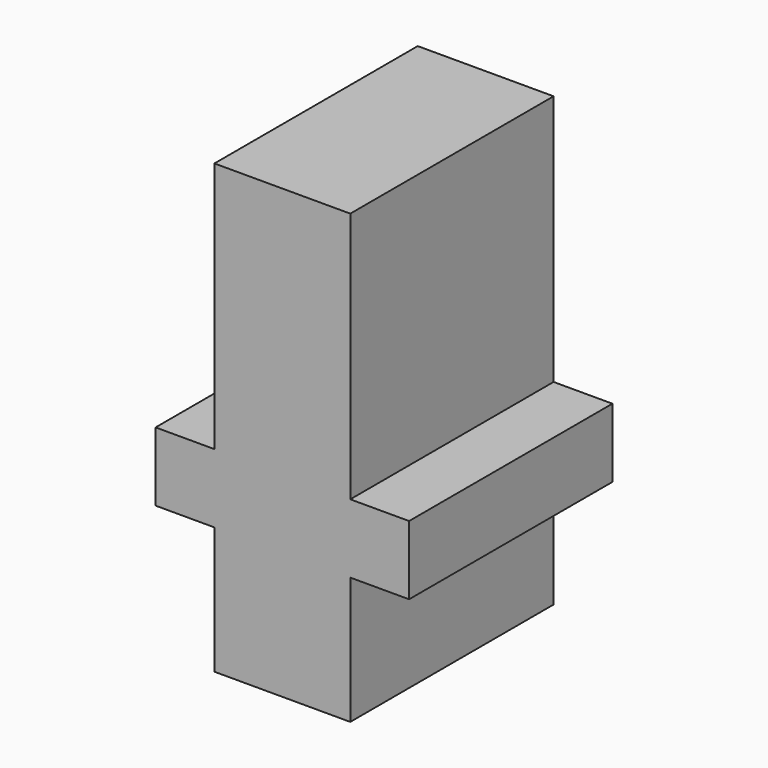
from build123d import *

# Parameters (mm, degrees)
F2_DEPTH = 4.7752


# Not quite as in the source:
# - a variable given as a bare number and used for a length is read in inches; the dataset says mm whatever the document's units were


with BuildPart() as f2:
    # F1 (on Front) → F2 (new body, symmetric)
    with BuildSketch(Plane.XZ):
        Polygon((-2.5527, 9.4505768009), (-2.5527, 0), (-4.7625, 0), (-4.7625, -2.5890231991), (-2.5527, -2.5890231991), (-2.5527, -7.3642231991), (2.5527, -7.3642231991), (2.5527, -2.5890231991), (4.7625, -2.5890231991), (4.7625, 0), (2.5527, 0), (2.5527, 9.4505768009), align=None)
    extrude(amount=F2_DEPTH, both=True)


solid = f2.part
